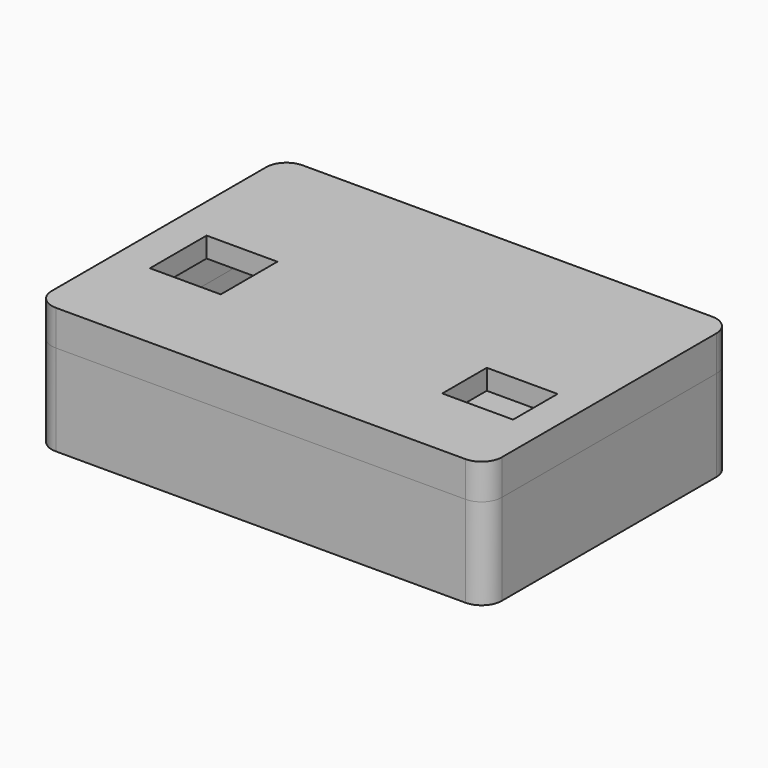
from build123d import *

# Parameters (mm, degrees)
F0_W      = 44.5
F0_H      = 30.5
F1_DEPTH  = 7
F2_T      = -2
F3_DEPTH  = 5.5
F4_T      = -2
F6_DEPTH  = 2
F5_W      = 0.8
F5_H      = 2
F9_R      = 2
F9_R_2    = 1
F10_DEPTH = 5
F11_W     = 7
F11_H     = 7
F11_H_2   = 5.5
F12_DEPTH = 2
F13_R     = 2
F13_2_R   = 2
F14_W     = 5.5
F14_H     = 2
F15_DEPTH = 2


with BuildPart() as f1:
    # F0 (on Top) → F1 (new body)
    with BuildSketch(Plane.XY):
        Rectangle(F0_W, F0_H)
    extrude(amount=-F1_DEPTH)

    # F2
    f2_openings = [f1.faces().sort_by_distance(p)[0] for p in [
        (0, 0, 0),
    ]]
    offset(amount=F2_T, openings=f2_openings)

    # F8: sweep along a path in F0
    with BuildLine(Plane.XY) as f8_path:
        Line((22.25, -15.25), (-22.25, -15.25))
        Line((-22.25, -15.25), (-22.25, 15.25))
        Line((-22.25, 15.25), (22.25, 15.25))
        Line((22.25, 15.25), (22.25, -15.25))
    # F5 (on Right) → F8 (sweep)
    with BuildSketch(Plane.YZ):
        with Locations((-14.85, 1)):
            Rectangle(F5_W, F5_H)
    sweep(path=f8_path.line, transition=Transition.RIGHT)

    # F9 (on face) → F10 (join)
    with BuildSketch(Plane.XY.offset(-5)):
        with Locations((0, -2.05)):
            Circle(F9_R)
        with Locations((0, -2.05)):
            Circle(F9_R_2, mode=Mode.SUBTRACT)
        with Locations((-16.5, -9.55)):
            Circle(F9_R)
        with Locations((-16.5, -9.55)):
            Circle(F9_R_2, mode=Mode.SUBTRACT)
        with Locations((16.5, 5.45)):
            Circle(F9_R)
        with Locations((16.5, 5.45)):
            Circle(F9_R_2, mode=Mode.SUBTRACT)
    extrude(amount=F10_DEPTH)

    # F13
    f13_edges = [f1.edges().sort_by_distance(p)[0] for p in [
        (22.25, 15.25, -2.5),
        (22.25, -15.25, -2.5),
        (-22.25, -15.25, -2.5),
        (-22.25, 15.25, -2.5),
    ]]
    fillet(f13_edges, radius=F13_R)


with BuildPart() as f3:
    # F0 (on Top) → F3 (new body)
    with BuildSketch(Plane.XY):
        Rectangle(F0_W, F0_H)
    extrude(amount=F3_DEPTH)

    # F4
    f4_openings = [f3.faces().sort_by_distance(p)[0] for p in [
        (0, 0, 0),
    ]]
    offset(amount=F4_T, openings=f4_openings)

    # F0 (on Top) → F6 (cut)
    with BuildSketch(Plane.XY):
        Rectangle(F0_W, F0_H)
    extrude(amount=F6_DEPTH, mode=Mode.SUBTRACT)

    # F7: sweep along a path in F7_path
    with BuildLine(Plane(origin=(20.25, -13.25, 2), x_dir=(0, 1, 0), z_dir=(0, 0, 1))) as f7_path:
        Line((0, 0), (0, 40.5))
        Line((0, 40.5), (26.5, 40.5))
        Line((26.5, 40.5), (26.5, 0))
        Line((26.5, 0), (0, 0))
    # F5 (on Right) → F7 (sweep)
    with BuildSketch(Plane.YZ):
        with Locations((-13.65, 1)):
            Rectangle(F5_W, F5_H)
    sweep(path=f7_path.line, transition=Transition.RIGHT)

    # F11 (on face) → F12 (cut, through all)
    with BuildSketch(Plane.XY.offset(5.5)):
        with Locations((-15.2, -2.05)):
            Rectangle(F11_W, F11_H)
        with Locations((15.5, -5.05)):
            Rectangle(F11_W, F11_H_2)
    extrude(amount=-F12_DEPTH, mode=Mode.SUBTRACT)

    # F13#2
    f13_2_edges = [f3.edges().sort_by_distance(p)[0] for p in [
        (-22.25, -15.25, 3.75),
        (-22.25, 15.25, 3.75),
        (22.25, -15.25, 3.75),
        (22.25, 15.25, 3.75),
    ]]
    fillet(f13_2_edges, radius=F13_2_R)


with BuildPart() as f15_tool:
    # F14 (on face) → F15 (new body)
    with BuildSketch(Plane(origin=(0, 15.25, 0), x_dir=(-1, 0, 0), z_dir=(0, 1, 0))):
        with Locations((14.5, 1)):
            Rectangle(F14_W, F14_H)
    extrude(amount=-F15_DEPTH)


with BuildPart() as f1_1:
    add(f1.part)

    # F15: cut by f15_tool
    add(f15_tool.part, mode=Mode.SUBTRACT)


with BuildPart() as f3_1:
    add(f3.part)

    # F15: cut by f15_tool
    add(f15_tool.part, mode=Mode.SUBTRACT)


solid = Compound([f1_1.part, f3_1.part])
